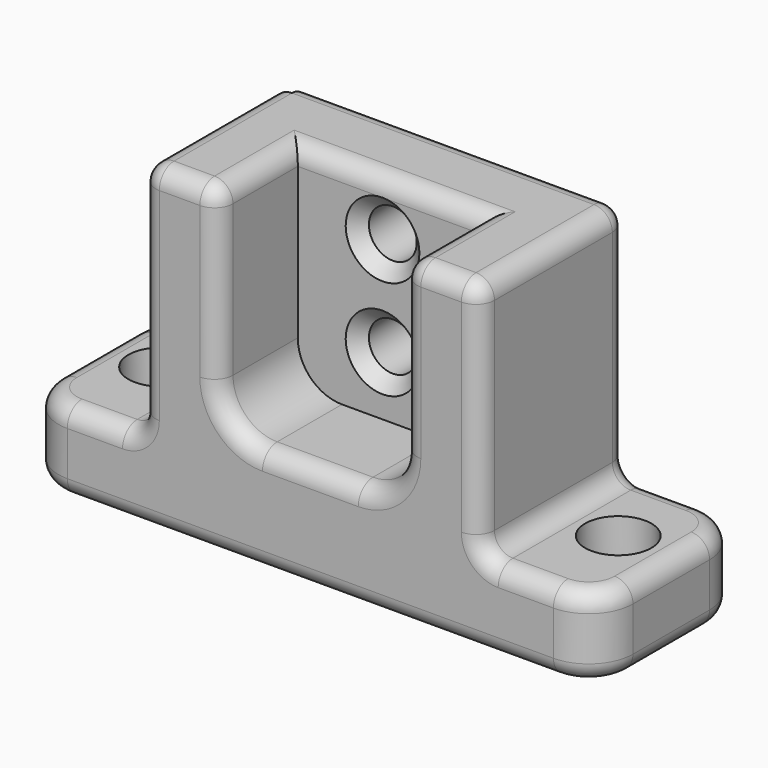
from build123d import *

# Parameters (mm, degrees)
F0_W           = 156
F0_H           = 50
F1_DEPTH       = 87
F2_W           = 32
F2_H           = 65
F3_DEPTH       = 50
F4_W           = 50
F4_H           = 58
F5_DEPTH       = 27
F7_D           = 13
F7_CBORE_D     = 18
F7_CBORE_DEPTH = 10
F9_D           = 13
F9_CSINK_D     = 20
F9_CSINK_ANGLE = 90
F10_R          = 12
F11_T1_DEPTH   = 50
F11_T3_DEPTH   = 75
F11_T5_DEPTH   = 28.5
F11_T7_DEPTH   = 22
F11_T9_DEPTH   = 50
F11_T11_DEPTH  = 28.5
F11_T13_DEPTH  = 117
F11_T15_DEPTH  = 132
F11_T17_DEPTH  = 41
F11_T19_DEPTH  = 26
F11_T21_DEPTH  = 26
F11_S25_W      = 5
F11_S25_H      = 5
F11_T26_DEPTH  = 5
F11_S31_W      = 5
F11_S31_H      = 5
F11_T32_DEPTH  = 5
F11_T36_ANGLE  = 90
F11_T38_ANGLE  = 90
F11_T40_ANGLE  = 90
F11_T42_ANGLE  = 90
F11_T44_ANGLE  = 90
F11_T46_ANGLE  = 90
F11_T51_DEPTH  = 34.5
F11_T55_DEPTH  = 62.5
F11_T62_DEPTH  = 62.5
F11_T66_DEPTH  = 34.5
F11_T69_DEPTH  = 15
F11_T71_DEPTH  = 15
F11_T73_DEPTH  = 55
F11_T75_DEPTH  = 26
F11_S79_W      = 5
F11_S79_H      = 5
F11_T80_DEPTH  = 5
F11_S85_W      = 5
F11_S85_H      = 5
F11_T86_DEPTH  = 5
F11_S91_W      = 5
F11_S91_H      = 5
F11_T92_DEPTH  = 5
F11_S97_W      = 5
F11_S97_H      = 5
F11_T98_DEPTH  = 5
F11_T102_ANGLE = 90
F11_T104_ANGLE = 90
F11_T106_ANGLE = 90
F11_T108_ANGLE = 90
F11_T110_ANGLE = 90
F11_T112_ANGLE = 90
F11_T114_ANGLE = 90
F11_T116_ANGLE = 90


# Not quite as in the source:
# - a fillet or chamfer that OpenCascade refuses, or shapes differently, is made with other operations: its cross-section is extruded or revolved along the edge and cut away or added


with BuildPart() as f1:
    # F0 (on Top) → F1 (new body)
    with BuildSketch(Plane.XY):
        with Locations((78, 25)):
            Rectangle(F0_W, F0_H)
    extrude(amount=F1_DEPTH)

    # F2 (on face) → F3 (cut, through all)
    with BuildSketch(Plane.XZ):
        with Locations((16, 54.5)):
            Rectangle(F2_W, F2_H)
        with Locations((140, 54.5)):
            Rectangle(F2_W, F2_H)
    extrude(amount=-F3_DEPTH, mode=Mode.SUBTRACT)

    # F4 (on face) → F5 (cut)
    with BuildSketch(Plane.XZ):
        with Locations((78, 58)):
            Rectangle(F4_W, F4_H)
    extrude(amount=-F5_DEPTH, mode=Mode.SUBTRACT)

    # F7 (through all)
    with Locations(Plane.XY.offset(22)):
        with Locations((16, 27), (140, 27)):
            CounterBoreHole(F7_D / 2, F7_CBORE_D / 2, F7_CBORE_DEPTH)

    # F9 (through all)
    with Locations(Plane.XZ.offset(-27)):
        with Locations((76, 72), (76, 45)):
            CounterSinkHole(F9_D / 2, F9_CSINK_D / 2, counter_sink_angle=F9_CSINK_ANGLE)

    # F10
    f10_edges = [f1.edges().sort_by_distance(p)[0] for p in [
        (156, 0, 11),
        (156, 50, 11),
        (103, 13.5, 29),
        (53, 13.5, 29),
        (0, 50, 11),
        (0, 0, 11),
    ]]
    fillet(f10_edges, radius=F10_R)

    # F11: fillet of radius 5 on 37 edges, made by hand

    # F11_s2 → F11_t1 (join)
    with BuildSketch(Plane.XZ.offset(-50)):
        with BuildLine():
            ThreePointArc((129, 22), (125.4644660941, 23.4644660941), (124, 27))
            Line((124, 27), (124, 22))
            Line((124, 22), (129, 22))
        make_face()
        with BuildLine():
            ThreePointArc((27, 22), (30.5355339059, 23.4644660941), (32, 27))
            Line((32, 27), (32, 22))
            Line((32, 22), (27, 22))
        make_face()
    extrude(amount=F11_T1_DEPTH)

    # F11_s4 → F11_t3 (cut)
    with BuildSketch(Plane.XZ.offset(-62.5)):
        with BuildLine():
            ThreePointArc((124, 82), (122.5355339059, 85.5355339059), (119, 87))
            Line((119, 87), (124, 87))
            Line((124, 87), (124, 82))
        make_face()
        with BuildLine():
            ThreePointArc((32, 82), (33.4644660941, 85.5355339059), (37, 87))
            Line((37, 87), (32, 87))
            Line((32, 87), (32, 82))
        make_face()
    extrude(amount=F11_T3_DEPTH, mode=Mode.SUBTRACT)

    # F11_s6 → F11_t5 (cut)
    with BuildSketch(Plane.YZ.offset(108)):
        with BuildLine():
            ThreePointArc((0, 82), (1.4644660941, 85.5355339059), (5, 87))
            Line((5, 87), (0, 87))
            Line((0, 87), (0, 82))
        make_face()
    extrude(amount=F11_T5_DEPTH, mode=Mode.SUBTRACT)

    # F11_s8 → F11_t7 (cut)
    with BuildSketch(Plane.XZ.offset(-27)):
        with BuildLine():
            ThreePointArc((108, 87), (104.4644660941, 85.5355339059), (103, 82))
            Line((103, 82), (103, 87))
            Line((103, 87), (108, 87))
        make_face()
        with BuildLine():
            ThreePointArc((48, 87), (51.5355339059, 85.5355339059), (53, 82))
            Line((53, 82), (53, 87))
            Line((53, 87), (48, 87))
        make_face()
    extrude(amount=F11_T7_DEPTH, mode=Mode.SUBTRACT)

    # F11_s10 → F11_t9 (cut)
    with BuildSketch(Plane.YZ.offset(53)):
        with BuildLine():
            ThreePointArc((32, 87), (28.4644660941, 85.5355339059), (27, 82))
            Line((27, 82), (27, 87))
            Line((27, 87), (32, 87))
        make_face()
    extrude(amount=F11_T9_DEPTH, mode=Mode.SUBTRACT)

    # F11_s12 → F11_t11 (cut)
    with BuildSketch(Plane.YZ.offset(19.5)):
        with BuildLine():
            ThreePointArc((0, 82), (1.4644660941, 85.5355339059), (5, 87))
            Line((5, 87), (0, 87))
            Line((0, 87), (0, 82))
        make_face()
    extrude(amount=F11_T11_DEPTH, mode=Mode.SUBTRACT)

    # F11_s14 → F11_t13 (cut)
    with BuildSketch(Plane.YZ.offset(19.5)):
        with BuildLine():
            ThreePointArc((50, 82), (48.5355339059, 85.5355339059), (45, 87))
            Line((45, 87), (50, 87))
            Line((50, 87), (50, 82))
        make_face()
    extrude(amount=F11_T13_DEPTH, mode=Mode.SUBTRACT)

    # F11_s16 → F11_t15 (cut)
    with BuildSketch(Plane.YZ.offset(12)):
        with BuildLine():
            ThreePointArc((5, 0), (1.4644660941, 1.4644660941), (0, 5))
            Line((0, 5), (0, 0))
            Line((0, 0), (5, 0))
        make_face()
        with BuildLine():
            ThreePointArc((45, 0), (48.5355339059, 1.4644660941), (50, 5))
            Line((50, 5), (50, 0))
            Line((50, 0), (45, 0))
        make_face()
    extrude(amount=F11_T15_DEPTH, mode=Mode.SUBTRACT)

    # F11_s18 → F11_t17 (cut)
    with BuildSketch(Plane.XY.offset(41)):
        with BuildLine():
            ThreePointArc((48, 0), (51.5355339059, 1.4644660941), (53, 5))
            Line((53, 5), (53, 0))
            Line((53, 0), (48, 0))
        make_face()
        with BuildLine():
            ThreePointArc((108, 0), (104.4644660941, 1.4644660941), (103, 5))
            Line((103, 5), (103, 0))
            Line((103, 0), (108, 0))
        make_face()
    extrude(amount=F11_T17_DEPTH, mode=Mode.SUBTRACT)

    # F11_s20 → F11_t19 (cut)
    with BuildSketch(Plane.YZ.offset(65)):
        with BuildLine():
            ThreePointArc((0, 24), (1.4644660941, 27.5355339059), (5, 29))
            Line((5, 29), (0, 29))
            Line((0, 29), (0, 24))
        make_face()
    extrude(amount=F11_T19_DEPTH, mode=Mode.SUBTRACT)

    # F11_s22 → F11_t21 (cut)
    with BuildSketch(Plane.XZ.offset(-38)):
        with BuildLine():
            ThreePointArc((0, 5), (1.4644660941, 1.4644660941), (5, 0))
            Line((5, 0), (0, 0))
            Line((0, 0), (0, 5))
        make_face()
        with BuildLine():
            ThreePointArc((151, 0), (154.5355339059, 1.4644660941), (156, 5))
            Line((156, 5), (156, 0))
            Line((156, 0), (151, 0))
        make_face()
    extrude(amount=F11_T21_DEPTH, mode=Mode.SUBTRACT)


with BuildPart() as f11_tool24:
    # F11_s25 → F11_t26 (new body)
    with BuildSketch(Plane.XY.offset(82)):
        with Locations((105.5, 2.5)):
            Rectangle(F11_S25_W, F11_S25_H)
    extrude(amount=F11_T26_DEPTH)

    # F11_s27 → F11_t28 (revolve, cut)
    with BuildSketch(Plane(origin=(108, 5, 82), x_dir=(0.7071067812, 0.7071067812, 0), z_dir=(0.7071067812, -0.7071067812, 0))):
        with BuildLine():
            ThreePointArc((0, -5), (5, 0), (0, 5))
            Line((0, 5), (0, -5))
        make_face()
    revolve(axis=Axis((108, 5, 82), (0, 0, 1)), mode=Mode.SUBTRACT)


with BuildPart() as f1_1:
    add(f1.part)

    # F11_t23: cut F11_tool24
    add(f11_tool24.part, mode=Mode.SUBTRACT)


with BuildPart() as f11_tool30:
    # F11_s31 → F11_t32 (new body)
    with BuildSketch(Plane.XY.offset(82)):
        with Locations((50.5, 2.5)):
            Rectangle(F11_S31_W, F11_S31_H)
    extrude(amount=F11_T32_DEPTH)

    # F11_s33 → F11_t34 (revolve, cut)
    with BuildSketch(Plane(origin=(48, 5, 82), x_dir=(-0.7071067812, 0.7071067812, 0), z_dir=(0.7071067812, 0.7071067812, 0))):
        with BuildLine():
            ThreePointArc((0, -5), (5, 0), (0, 5))
            Line((0, 5), (0, -5))
        make_face()
    revolve(axis=Axis((48, 5, 82), (0, 0, 1)), mode=Mode.SUBTRACT)


with BuildPart() as f1_2:
    add(f1_1.part)

    # F11_t29: cut F11_tool30
    add(f11_tool30.part, mode=Mode.SUBTRACT)

    # F11_s35 → F11_t36 (revolve, cut)
    with BuildSketch(Plane.YZ.offset(65)):
        with BuildLine():
            ThreePointArc((0, 24), (1.4644660941, 27.5355339059), (5, 29))
            Line((5, 29), (0, 29))
            Line((0, 29), (0, 24))
        make_face()
    revolve(axis=Axis((65, 0, 41), (0, 1, 0)), revolution_arc=F11_T36_ANGLE, mode=Mode.SUBTRACT)

    # F11_s37 → F11_t38 (revolve, cut)
    with BuildSketch(Plane.XY.offset(41)):
        with BuildLine():
            ThreePointArc((108, 0), (104.4644660941, 1.4644660941), (103, 5))
            Line((103, 5), (103, 0))
            Line((103, 0), (108, 0))
        make_face()
    revolve(axis=Axis((91, 0, 41), (0, 1, 0)), revolution_arc=F11_T38_ANGLE, mode=Mode.SUBTRACT)

    # F11_s39 → F11_t40 (revolve, cut)
    with BuildSketch(Plane.XZ.offset(-38)):
        with BuildLine():
            ThreePointArc((5, 0), (1.4644660941, 1.4644660941), (0, 5))
            Line((0, 5), (0, 0))
            Line((0, 0), (5, 0))
        make_face()
    revolve(axis=Axis((12, 38, 0), (0, 0, -1)), revolution_arc=F11_T40_ANGLE, mode=Mode.SUBTRACT)

    # F11_s41 → F11_t42 (revolve, cut)
    with BuildSketch(Plane.XZ.offset(-12)):
        with BuildLine():
            ThreePointArc((5, 0), (1.4644660941, 1.4644660941), (0, 5))
            Line((0, 5), (0, 0))
            Line((0, 0), (5, 0))
        make_face()
    revolve(axis=Axis((12, 12, 0), (0, 0, 1)), revolution_arc=F11_T42_ANGLE, mode=Mode.SUBTRACT)

    # F11_s43 → F11_t44 (revolve, cut)
    with BuildSketch(Plane.YZ.offset(144)):
        with BuildLine():
            ThreePointArc((45, 0), (48.5355339059, 1.4644660941), (50, 5))
            Line((50, 5), (50, 0))
            Line((50, 0), (45, 0))
        make_face()
    revolve(axis=Axis((144, 38, 0), (0, 0, -1)), revolution_arc=F11_T44_ANGLE, mode=Mode.SUBTRACT)

    # F11_s45 → F11_t46 (revolve, cut)
    with BuildSketch(Plane.YZ.offset(144)):
        with BuildLine():
            ThreePointArc((5, 0), (1.4644660941, 1.4644660941), (0, 5))
            Line((0, 5), (0, 0))
            Line((0, 0), (5, 0))
        make_face()
    revolve(axis=Axis((144, 12, 0), (0, 0, 1)), revolution_arc=F11_T46_ANGLE, mode=Mode.SUBTRACT)


with BuildPart() as f11_tool49:
    # F11_s50 → F11_t51 (new body)
    with BuildSketch(Plane.XZ.offset(-5)):
        with BuildLine():
            ThreePointArc((108, 87), (104.4644660941, 85.5355339059), (103, 82))
            Line((103, 82), (103, 87))
            Line((103, 87), (108, 87))
        make_face()
    extrude(amount=-F11_T51_DEPTH)

    split(bisect_by=Plane.XZ.offset(-27), keep=Keep.BOTTOM)


with BuildPart() as f11_tool53:
    # F11_s54 → F11_t55 (new body)
    with BuildSketch(Plane.YZ.offset(115.5)):
        with BuildLine():
            ThreePointArc((32, 87), (28.4644660941, 85.5355339059), (27, 82))
            Line((27, 82), (27, 87))
            Line((27, 87), (32, 87))
        make_face()
    extrude(amount=-F11_T55_DEPTH)

    split(bisect_by=Plane.YZ.offset(103), keep=Keep.TOP)


with BuildPart() as f11_tool49_1:
    add(f11_tool49.part)

    # F11_t57: intersect F11_tool53
    add(f11_tool53.part, mode=Mode.INTERSECT)


with BuildPart() as f1_3:
    add(f1_2.part)

    # F11_t47: cut F11_tool49
    add(f11_tool49_1.part, mode=Mode.SUBTRACT)


with BuildPart() as f11_tool60:
    # F11_s61 → F11_t62 (new body)
    with BuildSketch(Plane.YZ.offset(103)):
        with BuildLine():
            ThreePointArc((32, 87), (28.4644660941, 85.5355339059), (27, 82))
            Line((27, 82), (27, 87))
            Line((27, 87), (32, 87))
        make_face()
    extrude(amount=-F11_T62_DEPTH)

    split(bisect_by=Plane.YZ.offset(53), keep=Keep.BOTTOM)


with BuildPart() as f11_tool64:
    # F11_s65 → F11_t66 (new body)
    with BuildSketch(Plane.XZ.offset(-5)):
        with BuildLine():
            ThreePointArc((48, 87), (51.5355339059, 85.5355339059), (53, 82))
            Line((53, 82), (53, 87))
            Line((53, 87), (48, 87))
        make_face()
    extrude(amount=-F11_T66_DEPTH)

    split(bisect_by=Plane.XZ.offset(-27), keep=Keep.BOTTOM)


with BuildPart() as f11_tool60_1:
    add(f11_tool60.part)

    # F11_t68: intersect F11_tool64
    add(f11_tool64.part, mode=Mode.INTERSECT)


with BuildPart() as f1_4:
    add(f1_3.part)

    # F11_t58: cut F11_tool60
    add(f11_tool60_1.part, mode=Mode.SUBTRACT)

    # F11_s70 → F11_t69 (cut)
    with BuildSketch(Plane.YZ.offset(12)):
        with BuildLine():
            ThreePointArc((0, 17), (1.4644660941, 20.5355339059), (5, 22))
            Line((5, 22), (0, 22))
            Line((0, 22), (0, 17))
        make_face()
        with BuildLine():
            ThreePointArc((50, 17), (48.5355339059, 20.5355339059), (45, 22))
            Line((45, 22), (50, 22))
            Line((50, 22), (50, 17))
        make_face()
    extrude(amount=F11_T69_DEPTH, mode=Mode.SUBTRACT)

    # F11_s72 → F11_t71 (cut)
    with BuildSketch(Plane.YZ.offset(129)):
        with BuildLine():
            ThreePointArc((0, 17), (1.4644660941, 20.5355339059), (5, 22))
            Line((5, 22), (0, 22))
            Line((0, 22), (0, 17))
        make_face()
        with BuildLine():
            ThreePointArc((45, 22), (48.5355339059, 20.5355339059), (50, 17))
            Line((50, 17), (50, 22))
            Line((50, 22), (45, 22))
        make_face()
    extrude(amount=F11_T71_DEPTH, mode=Mode.SUBTRACT)

    # F11_s74 → F11_t73 (cut)
    with BuildSketch(Plane.XY.offset(27)):
        with BuildLine():
            ThreePointArc((37, 0), (33.4644660941, 1.4644660941), (32, 5))
            Line((32, 5), (32, 0))
            Line((32, 0), (37, 0))
        make_face()
        with BuildLine():
            ThreePointArc((119, 0), (122.5355339059, 1.4644660941), (124, 5))
            Line((124, 5), (124, 0))
            Line((124, 0), (119, 0))
        make_face()
        with BuildLine():
            ThreePointArc((124, 45), (122.5355339059, 48.5355339059), (119, 50))
            Line((119, 50), (124, 50))
            Line((124, 50), (124, 45))
        make_face()
        with BuildLine():
            ThreePointArc((32, 45), (33.4644660941, 48.5355339059), (37, 50))
            Line((37, 50), (32, 50))
            Line((32, 50), (32, 45))
        make_face()
    extrude(amount=F11_T73_DEPTH, mode=Mode.SUBTRACT)

    # F11_s76 → F11_t75 (cut)
    with BuildSketch(Plane.XZ.offset(-38)):
        with BuildLine():
            ThreePointArc((0, 17), (1.4644660941, 20.5355339059), (5, 22))
            Line((5, 22), (0, 22))
            Line((0, 22), (0, 17))
        make_face()
        with BuildLine():
            ThreePointArc((151, 22), (154.5355339059, 20.5355339059), (156, 17))
            Line((156, 17), (156, 22))
            Line((156, 22), (151, 22))
        make_face()
    extrude(amount=F11_T75_DEPTH, mode=Mode.SUBTRACT)


with BuildPart() as f11_tool78:
    # F11_s79 → F11_t80 (new body)
    with BuildSketch(Plane.YZ.offset(37)):
        with Locations((47.5, 84.5)):
            Rectangle(F11_S79_W, F11_S79_H)
    extrude(amount=-F11_T80_DEPTH)

    # F11_s81 → F11_t82 (revolve, cut)
    with BuildSketch(Plane(origin=(37, 45, 82), x_dir=(0, -0.7071067812, -0.7071067812), z_dir=(0, 0.7071067812, -0.7071067812))):
        with BuildLine():
            ThreePointArc((0, -5), (5, 0), (0, 5))
            Line((0, 5), (0, -5))
        make_face()
    revolve(axis=Axis((37, 45, 82), (-1, 0, 0)), mode=Mode.SUBTRACT)


with BuildPart() as f1_5:
    add(f1_4.part)

    # F11_t77: cut F11_tool78
    add(f11_tool78.part, mode=Mode.SUBTRACT)


with BuildPart() as f11_tool84:
    # F11_s85 → F11_t86 (new body)
    with BuildSketch(Plane.YZ.offset(119)):
        with Locations((47.5, 84.5)):
            Rectangle(F11_S85_W, F11_S85_H)
    extrude(amount=F11_T86_DEPTH)

    # F11_s87 → F11_t88 (revolve, cut)
    with BuildSketch(Plane(origin=(119, 45, 82), x_dir=(0, -0.7071067812, -0.7071067812), z_dir=(0, -0.7071067812, 0.7071067812))):
        with BuildLine():
            ThreePointArc((0, -5), (5, 0), (0, 5))
            Line((0, 5), (0, -5))
        make_face()
    revolve(axis=Axis((119, 45, 82), (1, 0, 0)), mode=Mode.SUBTRACT)


with BuildPart() as f1_6:
    add(f1_5.part)

    # F11_t83: cut F11_tool84
    add(f11_tool84.part, mode=Mode.SUBTRACT)


with BuildPart() as f11_tool90:
    # F11_s91 → F11_t92 (new body)
    with BuildSketch(Plane.XZ.offset(-5)):
        with Locations((121.5, 84.5)):
            Rectangle(F11_S91_W, F11_S91_H)
    extrude(amount=F11_T92_DEPTH)

    # F11_s93 → F11_t94 (revolve, cut)
    with BuildSketch(Plane(origin=(119, 5, 82), x_dir=(-0.7071067812, 0, -0.7071067812), z_dir=(-0.7071067812, 0, 0.7071067812))):
        with BuildLine():
            ThreePointArc((0, -5), (5, 0), (0, 5))
            Line((0, 5), (0, -5))
        make_face()
    revolve(axis=Axis((119, 5, 82), (0, -1, 0)), mode=Mode.SUBTRACT)


with BuildPart() as f1_7:
    add(f1_6.part)

    # F11_t89: cut F11_tool90
    add(f11_tool90.part, mode=Mode.SUBTRACT)


with BuildPart() as f11_tool96:
    # F11_s97 → F11_t98 (new body)
    with BuildSketch(Plane.XZ.offset(-5)):
        with Locations((34.5, 84.5)):
            Rectangle(F11_S97_W, F11_S97_H)
    extrude(amount=F11_T98_DEPTH)

    # F11_s99 → F11_t100 (revolve, cut)
    with BuildSketch(Plane(origin=(37, 5, 82), x_dir=(0.7071067812, 0, -0.7071067812), z_dir=(-0.7071067812, 0, -0.7071067812))):
        with BuildLine():
            ThreePointArc((0, -5), (5, 0), (0, 5))
            Line((0, 5), (0, -5))
        make_face()
    revolve(axis=Axis((37, 5, 82), (0, -1, 0)), mode=Mode.SUBTRACT)


with BuildPart() as f1_8:
    add(f1_7.part)

    # F11_t95: cut F11_tool96
    add(f11_tool96.part, mode=Mode.SUBTRACT)

    # F11_s101 → F11_t102 (revolve, cut)
    with BuildSketch(Plane.XZ.offset(-38)):
        with BuildLine():
            ThreePointArc((0, 17), (1.4644660941, 20.5355339059), (5, 22))
            Line((5, 22), (0, 22))
            Line((0, 22), (0, 17))
        make_face()
    revolve(axis=Axis((12, 38, 22), (0, 0, -1)), revolution_arc=F11_T102_ANGLE, mode=Mode.SUBTRACT)

    # F11_s103 → F11_t104 (revolve, cut)
    with BuildSketch(Plane.XZ.offset(-12)):
        with BuildLine():
            ThreePointArc((5, 22), (1.4644660941, 20.5355339059), (0, 17))
            Line((0, 17), (0, 22))
            Line((0, 22), (5, 22))
        make_face()
    revolve(axis=Axis((12, 12, 22), (0, 0, 1)), revolution_arc=F11_T104_ANGLE, mode=Mode.SUBTRACT)

    # F11_s105 → F11_t106 (revolve, cut)
    with BuildSketch(Plane.YZ.offset(144)):
        with BuildLine():
            ThreePointArc((45, 22), (48.5355339059, 20.5355339059), (50, 17))
            Line((50, 17), (50, 22))
            Line((50, 22), (45, 22))
        make_face()
    revolve(axis=Axis((144, 38, 22), (0, 0, -1)), revolution_arc=F11_T106_ANGLE, mode=Mode.SUBTRACT)

    # F11_s107 → F11_t108 (revolve, cut)
    with BuildSketch(Plane.YZ.offset(144)):
        with BuildLine():
            ThreePointArc((5, 22), (1.4644660941, 20.5355339059), (0, 17))
            Line((0, 17), (0, 22))
            Line((0, 22), (5, 22))
        make_face()
    revolve(axis=Axis((144, 12, 22), (0, 0, 1)), revolution_arc=F11_T108_ANGLE, mode=Mode.SUBTRACT)

    # F11_s109 → F11_t110 (revolve, cut)
    with BuildSketch(Plane.YZ.offset(27)):
        with BuildLine():
            ThreePointArc((45, 22), (48.5355339059, 20.5355339059), (50, 17))
            Line((50, 17), (50, 22))
            Line((50, 22), (45, 22))
        make_face()
    revolve(axis=Axis((27, 50, 27), (0, -1, 0)), revolution_arc=F11_T110_ANGLE, mode=Mode.SUBTRACT)

    # F11_s111 → F11_t112 (revolve, cut)
    with BuildSketch(Plane.YZ.offset(129)):
        with BuildLine():
            ThreePointArc((45, 22), (48.5355339059, 20.5355339059), (50, 17))
            Line((50, 17), (50, 22))
            Line((50, 22), (45, 22))
        make_face()
    revolve(axis=Axis((129, 50, 27), (0, 1, 0)), revolution_arc=F11_T112_ANGLE, mode=Mode.SUBTRACT)

    # F11_s113 → F11_t114 (revolve, cut)
    with BuildSketch(Plane.YZ.offset(129)):
        with BuildLine():
            ThreePointArc((0, 17), (1.4644660941, 20.5355339059), (5, 22))
            Line((5, 22), (0, 22))
            Line((0, 22), (0, 17))
        make_face()
    revolve(axis=Axis((129, 0, 27), (0, 1, 0)), revolution_arc=F11_T114_ANGLE, mode=Mode.SUBTRACT)

    # F11_s115 → F11_t116 (revolve, cut)
    with BuildSketch(Plane.YZ.offset(27)):
        with BuildLine():
            ThreePointArc((0, 17), (1.4644660941, 20.5355339059), (5, 22))
            Line((5, 22), (0, 22))
            Line((0, 22), (0, 17))
        make_face()
    revolve(axis=Axis((27, 0, 27), (0, -1, 0)), revolution_arc=F11_T116_ANGLE, mode=Mode.SUBTRACT)


solid = f1_8.part
